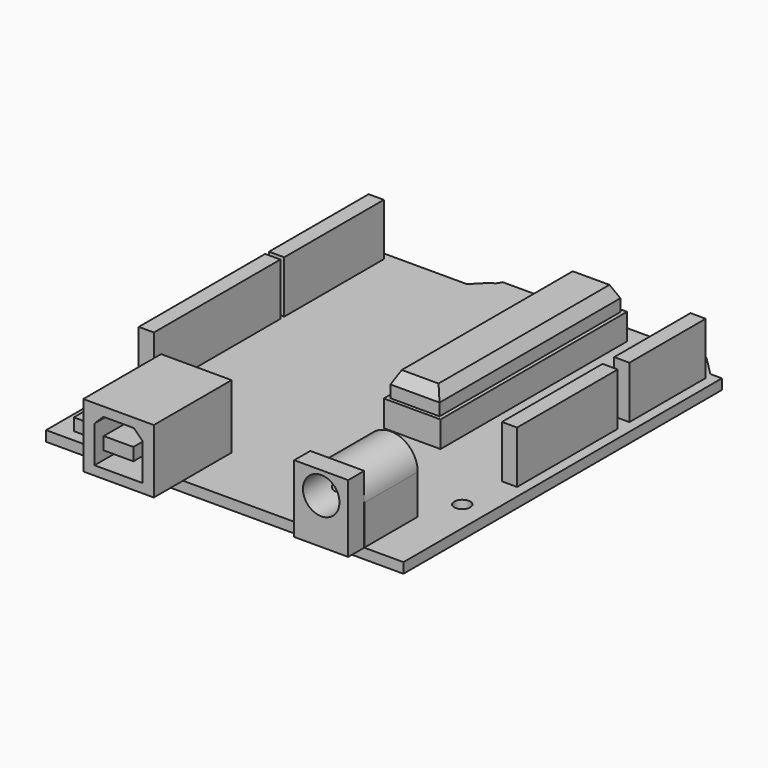
from build123d import *

# Parameters (mm, degrees)
F1_DEPTH   = 1.69
F2_W       = 2.5
F2_H       = 20.7
F3_DEPTH   = 8.6
F2_H_2     = 15.69
F2_H_3     = 20.481327492
F2_H_4     = 26
F6_DEPTH   = 11
F7_W       = 8.87868274
F7_H       = 11.1249446636
F8_DEPTH   = 3.3
F9_R       = 3
F10_DEPTH  = 12.8
F11_R      = 0.5
F12_DEPTH  = 10
F13_W      = 11.6
F13_H      = 10
F14_DEPTH  = 10.5
F15_W      = 11.6
F15_H      = 10.5
F16_DEPTH  = 6
F18_DEPTH  = 14.14393
F19_W      = 4.8785965383
F19_H      = 2.0820805803
F20_DEPTH  = 14.14393
F21_W      = 6.5
F21_H      = 6.5
F22_DEPTH  = 2
F23_R      = 2.2427667378
F24_DEPTH  = 1
F25_W      = 9.3276520822
F25_H      = 38.3693373368
F26_DEPTH  = 4.29568
F27_W      = 8.0811752376
F27_H      = 37.1907090231
F28_DEPTH  = 2
F30_W      = 6.0478351079
F30_H      = 35.1617564447
F28_FACE_W = 8.0811752376
F28_FACE_H = 37.1907090231
F33_DEPTH  = 1.691
F34_R      = 1.1
F34_R_2    = 1.3134018391
F35_DEPTH  = 1.691


# Not quite as in the source:
# - a feature of the source that left no trace in its solid (it failed there, or was rolled back) is left out


with BuildPart() as f1:
    # F0 (on Top) → F1 (new body)
    with BuildSketch(Plane.XY):
        Polygon((24.2, 34.4), (-9.2744298918, 34.4), (-12.5744298918, 31.1), (-29.4, 31.1), (-29.4, -34.4), (29.4, -34.4), (29.4, 31.1), (27.5, 31.1), align=None)
    extrude(amount=F1_DEPTH)

    # F32 (on face) → F33 (cut, through all)
    with BuildSketch(Plane.XY.offset(1.69)):
        with BuildLine():
            Line((-9.4422222306, 34.2322076612), (-10.3304163494, 33.3440135424))
            ThreePointArc((-10.3304163494, 33.3440135424), (-9.7470766516, 33.6488679634), (-9.4422222306, 34.2322076612))
        make_face()
        with BuildLine():
            ThreePointArc((-9.4422222306, 34.2322076612), (-9.4292347048, 34.3290613178), (-9.4248941109, 34.4266854227))
            ThreePointArc((-9.4248941109, 34.4266854227), (-11.3686729734, 35.132402952), (-10.3304163494, 33.3440135424))
            Line((-10.3304163494, 33.3440135424), (-9.4422222306, 34.2322076612))
        make_face()
        with BuildLine():
            Line((23.8030258555, 34.4), (21.6036733251, 34.4))
            ThreePointArc((21.6036733251, 34.4), (22.7033495903, 33.3266854227), (23.8030258555, 34.4))
        make_face()
        with BuildLine():
            ThreePointArc((23.8033495903, 34.4266854227), (22.6900058972, 35.526604486), (21.6036733251, 34.4))
            Line((21.6036733251, 34.4), (23.8030258555, 34.4))
            ThreePointArc((23.8030258555, 34.4), (23.8032686536, 34.4133417295), (23.8033495903, 34.4266854227))
        make_face()
    extrude(amount=-F33_DEPTH, mode=Mode.SUBTRACT)

    # F34 (on face) → F35 (cut, through all)
    with BuildSketch(Plane.XY.offset(1.69)):
        with Locations((-25.2349545183, -17.141347751)):
            Circle(F34_R)
        with Locations((25.2761915326, -17.141347751)):
            Circle(F34_R_2)
    extrude(amount=-F35_DEPTH, mode=Mode.SUBTRACT)


with BuildPart() as f3:
    # F2 (on face) → F3 (new body)
    with BuildSketch(Plane.XY.offset(1.69)):
        with Locations((26.48, 1.41)):
            Rectangle(F2_W, F2_H)
    extrude(amount=F3_DEPTH)


with BuildPart() as f3b:
    # F2 (on face) → F3, piece 2 (new body)
    with BuildSketch(Plane.XY.offset(1.69)):
        with Locations((26.48, 22.005)):
            Rectangle(F2_W, F2_H_2)
    extrude(amount=F3_DEPTH)


with BuildPart() as f3c:
    # F2 (on face) → F3, piece 3 (new body)
    with BuildSketch(Plane.XY.offset(1.69)):
        with Locations((-26.48, 19.609336254)):
            Rectangle(F2_W, F2_H_3)
    extrude(amount=F3_DEPTH)


with BuildPart() as f3d:
    # F2 (on face) → F3, piece 4 (new body)
    with BuildSketch(Plane.XY.offset(1.69)):
        with Locations((-26.48, -4.431327492)):
            Rectangle(F2_W, F2_H_4)
    extrude(amount=F3_DEPTH)


with BuildPart() as f6:
    # F5 (on offset) → F6 (new body)
    with BuildSketch(Plane.XZ.offset(34.4)):
        with BuildLine():
            Line((14.0722493033, 1.6842637178), (22.9522493033, 1.6842637178))
            Line((22.9522493033, 1.6842637178), (22.9522493033, 8.1842637178))
            ThreePointArc((22.9522493033, 8.1842637178), (18.5122493033, 12.6242637178), (14.0722493033, 8.1842637178))
            Line((14.0722493033, 8.1842637178), (14.0722493033, 1.6842637178))
        make_face()
    extrude(amount=-F6_DEPTH)

    # F7 (on offset) → F8 (join)
    with BuildSketch(Plane.XZ.offset(34.4)):
        with Locations((18.5108794831, 7.2514217463)):
            Rectangle(F7_W, F7_H)
    extrude(amount=F8_DEPTH)

    # F9 (on face) → F10 (cut)
    with BuildSketch(Plane.XZ.offset(37.7)):
        with Locations((18.5108794831, 9.124157019)):
            Circle(F9_R)
    extrude(amount=-F10_DEPTH, mode=Mode.SUBTRACT)


with BuildPart() as f12:
    # F11 (on face) → F12 (new body)
    with BuildSketch(Plane.XZ.offset(24.9)):
        with Locations((18.5108794831, 9.124157019)):
            Circle(F11_R)
    extrude(amount=F12_DEPTH)


with BuildPart() as f14:
    # F13 (on face) → F14 (new body)
    with BuildSketch(Plane.XY.offset(1.69)):
        with Locations((-12.6785661542, -29.4)):
            Rectangle(F13_W, F13_H)
    extrude(amount=F14_DEPTH)

    # F15 (on face) → F16 (join)
    with BuildSketch(Plane.XZ.offset(34.4)):
        with Locations((-12.6785661542, 6.94)):
            Rectangle(F15_W, F15_H)
    extrude(amount=F16_DEPTH)

    # F17 (on face) → F18 (cut)
    with BuildSketch(Plane.XZ.offset(40.4)):
        Polygon((-16.6285661542, 9.2491237447), (-16.6285661542, 3.19), (-8.7285661542, 3.19), (-8.7285661542, 9.2515923473), (-10.1669738069, 10.69), (-15.1876898989, 10.69), align=None)
    extrude(amount=-F18_DEPTH, mode=Mode.SUBTRACT)


with BuildPart() as f20:
    # F19 (on face) → F20 (new body, through all)
    with BuildSketch(Plane.XZ.offset(26.25607)):
        with Locations((-12.6773318529, 6.8805450574)):
            Rectangle(F19_W, F19_H)
    extrude(amount=F20_DEPTH)


with BuildPart() as f22:
    # F21 (on face) → F22 (new body)
    with BuildSketch(Plane.XY.offset(1.69)):
        with Locations((-23.1851451099, -29.143884778)):
            Rectangle(F21_W, F21_H)
    extrude(amount=F22_DEPTH)


with BuildPart() as f24:
    # F23 (on face) → F24 (new body)
    with BuildSketch(Plane.XY.offset(3.69)):
        with Locations((-23.1851451099, -29.143884778)):
            Circle(F23_R)
    extrude(amount=F24_DEPTH)


with BuildPart() as f26:
    # F25 (on face) → F26 (new body)
    with BuildSketch(Plane.XY.offset(1.69)):
        with Locations((8.8037233053, 12.316826851)):
            Rectangle(F25_W, F25_H)
    extrude(amount=F26_DEPTH)


with BuildPart() as f28:
    # F27 (on face) → F28 (new body)
    with BuildSketch(Plane.XY.offset(5.98568)):
        with Locations((8.8037233053, 12.316826851)):
            Rectangle(F27_W, F27_H)
    extrude(amount=F28_DEPTH)


with BuildPart() as f31:
    # F30 (on offset) → F31 section 0
    with BuildSketch(Plane.XY.offset(9.98568)):
        with Locations((8.8047666941, 12.3632361647)):
            Rectangle(F30_W, F30_H)
    # F28_face (on face) → F31 section 1
    with BuildSketch(Plane(origin=(8.8037233053, 12.316826851, 7.98568), x_dir=(1, 0, 0), z_dir=(0, 0, 1))):
        Rectangle(F28_FACE_W, F28_FACE_H)
    loft()


solid = Compound([f1.part, f3.part, f3b.part, f3c.part, f3d.part, f6.part, f12.part, f14.part, f20.part, f22.part, f24.part, f26.part, f28.part, f31.part])
